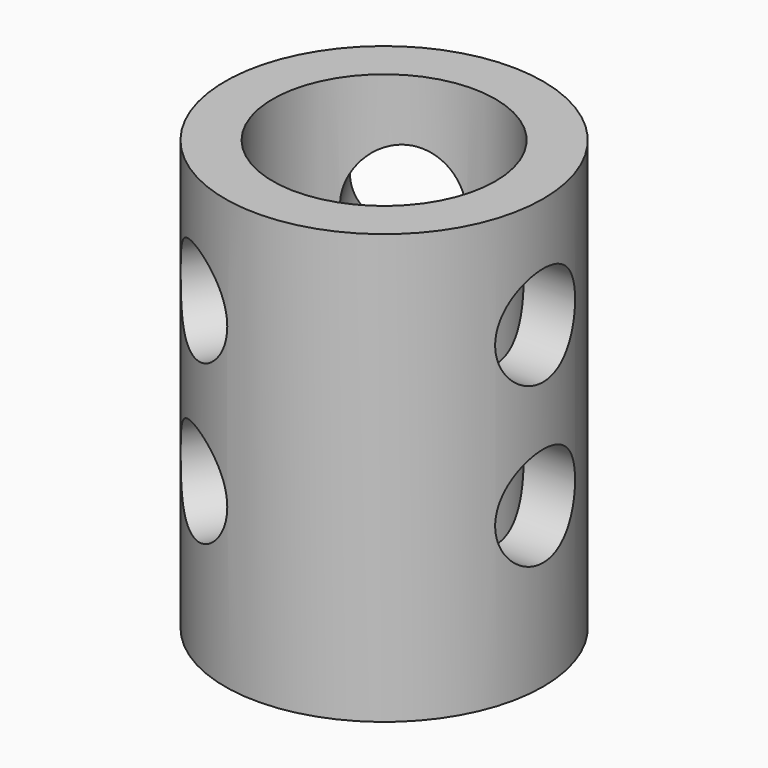
from build123d import *

# Parameters (mm, degrees)
F0_R       = 6.35
F0_R_2     = 2.159
F1_DEPTH   = 1.27
F2_R       = 6.35
F2_R_2     = 4.445
F3_DEPTH   = 15.875
F5_R       = 1.9939
F6_DEPTH   = 6.35
F7_COUNT   = 3
F8_R       = 1.9939
F6_FACE_R  = 1.9939
F9_DEPTH   = 6.35
F7_FACE_R  = 1.9939
F10_R      = 1.9939
F11_DEPTH  = 6.35
F7_FACE1_R = 1.9939
F12_R      = 1.9939
F13_DEPTH  = 6.35


with BuildPart() as f1:
    # F0 (on Top) → F1 (new body)
    with BuildSketch(Plane.XY):
        Circle(F0_R)
        Circle(F0_R_2, mode=Mode.SUBTRACT)
    extrude(amount=F1_DEPTH)

    # F2 (on face) → F3 (join)
    with BuildSketch(Plane.XY.offset(1.27)):
        Circle(F2_R)
        Circle(F2_R_2, mode=Mode.SUBTRACT)
    extrude(amount=F3_DEPTH)


with BuildPart() as f6:
    # F5 (on offset) → F6 (new body)
    with BuildSketch(Plane.YZ.offset(6.35)):
        with Locations((0, 6.35)):
            Circle(F5_R)
    extrude(amount=-F6_DEPTH)


with BuildPart() as f6b:
    # F5 (on offset) → F6, piece 2 (new body)
    with BuildSketch(Plane.YZ.offset(6.35)):
        with Locations((0, 12.7)):
            Circle(F5_R)
    extrude(amount=-F6_DEPTH)


with BuildPart() as f7_1:
    # F7: instance of F6
    add(f6.part.rotate(Axis((0, 0, 17.145), (0, 0, 1)), 1 * 360 / F7_COUNT))


with BuildPart() as f7_2:
    # F7: instance of F6
    add(f6.part.rotate(Axis((0, 0, 17.145), (0, 0, 1)), 2 * 360 / F7_COUNT))


with BuildPart() as f7_3:
    # F7: instance of F6b
    add(f6b.part.rotate(Axis((0, 0, 17.145), (0, 0, 1)), 1 * 360 / F7_COUNT))


with BuildPart() as f7_4:
    # F7: instance of F6b
    add(f6b.part.rotate(Axis((0, 0, 17.145), (0, 0, 1)), 2 * 360 / F7_COUNT))


with BuildPart() as f9_tool:
    # F8 (on face) + F6_face (on face) → F9 (new body)
    with BuildSketch(Plane.YZ.offset(6.35)):
        with Locations((0, 6.35)):
            Circle(F8_R)
    with BuildSketch(Plane(origin=(6.35, 0, 6.35), x_dir=(0, 1, 0), z_dir=(1, 0, 0))):
        with Locations((0, 6.35)):
            Circle(F6_FACE_R)
    extrude(amount=-F9_DEPTH)


with BuildPart() as f1_1:
    add(f1.part)

    # F9: cut by f9_tool
    add(f9_tool.part, mode=Mode.SUBTRACT)


with BuildPart() as f6_1:
    add(f6.part)

    # F9: cut by f9_tool
    add(f9_tool.part, mode=Mode.SUBTRACT)


with BuildPart() as f6b_1:
    add(f6b.part)

    # F9: cut by f9_tool
    add(f9_tool.part, mode=Mode.SUBTRACT)


with BuildPart() as f7_1_1:
    add(f7_1.part)

    # F9: cut by f9_tool
    add(f9_tool.part, mode=Mode.SUBTRACT)


with BuildPart() as f7_2_1:
    add(f7_2.part)

    # F9: cut by f9_tool
    add(f9_tool.part, mode=Mode.SUBTRACT)


with BuildPart() as f7_3_1:
    add(f7_3.part)

    # F9: cut by f9_tool
    add(f9_tool.part, mode=Mode.SUBTRACT)


with BuildPart() as f7_4_1:
    add(f7_4.part)

    # F9: cut by f9_tool
    add(f9_tool.part, mode=Mode.SUBTRACT)


with BuildPart() as f11_tool:
    # F7_face (on face) + F10 (on face) → F11 (new body)
    with BuildSketch(Plane(origin=(-3.175, 5.499261314, 6.35), x_dir=(-0.8660254038, -0.5, 0), z_dir=(-0.5, 0.8660254038, 0))):
        with Locations((0, 6.35)):
            Circle(F7_FACE_R)
    with BuildSketch(Plane(origin=(-3.175, 5.499261314, 0), x_dir=(-0.8660254038, -0.5, 0), z_dir=(-0.5, 0.8660254038, 0))):
        with Locations((0, 6.35)):
            Circle(F10_R)
    extrude(amount=-F11_DEPTH)


with BuildPart() as f1_2:
    add(f1_1.part)

    # F11: cut by f11_tool
    add(f11_tool.part, mode=Mode.SUBTRACT)


with BuildPart() as f7_1_2:
    add(f7_1_1.part)

    # F11: cut by f11_tool
    add(f11_tool.part, mode=Mode.SUBTRACT)


with BuildPart() as f7_2_2:
    add(f7_2_1.part)

    # F11: cut by f11_tool
    add(f11_tool.part, mode=Mode.SUBTRACT)


with BuildPart() as f7_3_2:
    add(f7_3_1.part)

    # F11: cut by f11_tool
    add(f11_tool.part, mode=Mode.SUBTRACT)


with BuildPart() as f7_4_2:
    add(f7_4_1.part)

    # F11: cut by f11_tool
    add(f11_tool.part, mode=Mode.SUBTRACT)


with BuildPart() as f13_tool:
    # F7_face1 (on face) + F12 (on face) → F13 (new body)
    with BuildSketch(Plane(origin=(-3.175, -5.499261314, 6.35), x_dir=(0.8660254038, -0.5, 0), z_dir=(-0.5, -0.8660254038, 0))):
        with Locations((0, 6.35)):
            Circle(F7_FACE1_R)
    with BuildSketch(Plane(origin=(-3.175, -5.499261314, 0), x_dir=(0.8660254038, -0.5, 0), z_dir=(-0.5, -0.8660254038, 0))):
        with Locations((0, 6.35)):
            Circle(F12_R)
    extrude(amount=-F13_DEPTH)


with BuildPart() as f1_3:
    add(f1_2.part)

    # F13: cut by f13_tool
    add(f13_tool.part, mode=Mode.SUBTRACT)


with BuildPart() as f7_2_3:
    add(f7_2_2.part)

    # F13: cut by f13_tool
    add(f13_tool.part, mode=Mode.SUBTRACT)


with BuildPart() as f7_4_3:
    add(f7_4_2.part)

    # F13: cut by f13_tool
    add(f13_tool.part, mode=Mode.SUBTRACT)


solid = f1_3.part
